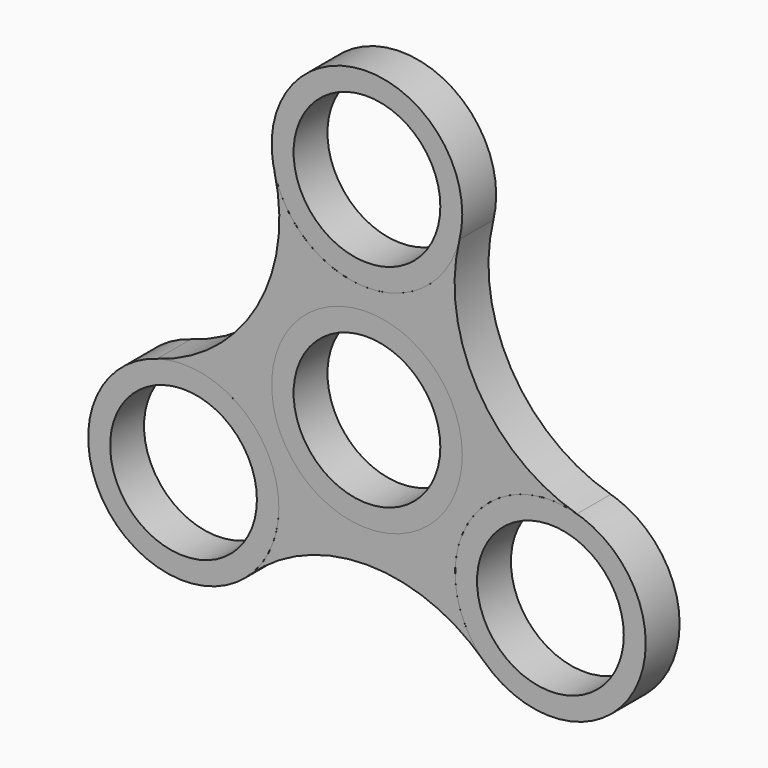
from build123d import *

# Parameters (mm, degrees)
F0_R     = 14.2875
F0_R_2   = 10.9982
F2_DEPTH = 6.35
F1_R     = 14.2875


with BuildPart() as f2:
    # F0 (on Front) → F2 (new body)
    with BuildSketch(Plane.XZ):
        with Locations((-27.4963065702, -15.875)):
            Circle(F0_R)
        with Locations((-27.4963065702, -15.875)):
            Circle(F0_R_2, mode=Mode.SUBTRACT)
    extrude(amount=F2_DEPTH)


with BuildPart() as f2b:
    # F0 (on Front) → F2, piece 2 (new body)
    with BuildSketch(Plane.XZ):
        Circle(F0_R)
        Circle(F0_R_2, mode=Mode.SUBTRACT)
    extrude(amount=F2_DEPTH)


with BuildPart() as f2c:
    # F0 (on Front) → F2, piece 3 (new body)
    with BuildSketch(Plane.XZ):
        with Locations((0, 31.75)):
            Circle(F0_R)
        with Locations((0, 31.75)):
            Circle(F0_R_2, mode=Mode.SUBTRACT)
    extrude(amount=F2_DEPTH)


with BuildPart() as f2d:
    # F0 (on Front) → F2, piece 4 (new body)
    with BuildSketch(Plane.XZ):
        with Locations((27.4963065702, -15.875)):
            Circle(F0_R)
        with Locations((27.4963065702, -15.875)):
            Circle(F0_R_2, mode=Mode.SUBTRACT)
    extrude(amount=F2_DEPTH)


with BuildPart() as f2e:
    # F1 (on Front) → F2, piece 5 (new body)
    with BuildSketch(Plane.XZ):
        with BuildLine():
            ThreePointArc((-13.8718760728, 28.3289313848), (-16.5359438351, 9.5470316245), (-31.4695122777, -2.1510686152))
            ThreePointArc((-31.4695122777, -2.1510686152), (-18.912441482, -4.4535326513), (-13.2088065702, -15.875))
            ThreePointArc((-13.2088065702, -15.875), (-14.3517276668, -21.4743483284), (-17.5976362049, -26.1778627696))
            ThreePointArc((-17.5976362049, -26.1778627696), (0, -19.094063249), (17.5976362049, -26.1778627696))
            ThreePointArc((17.5976362049, -26.1778627696), (15.1229686136, -8.73125), (31.4695122777, -2.1510686152))
            ThreePointArc((31.4695122777, -2.1510686152), (16.5359438351, 9.5470316245), (13.8718760728, 28.3289313848))
            ThreePointArc((13.8718760728, 28.3289313848), (0, 17.4625), (-13.8718760728, 28.3289313848))
        make_face()
        Circle(F1_R, mode=Mode.SUBTRACT)
    extrude(amount=F2_DEPTH)


solid = Compound([f2.part, f2b.part, f2c.part, f2d.part, f2e.part])
